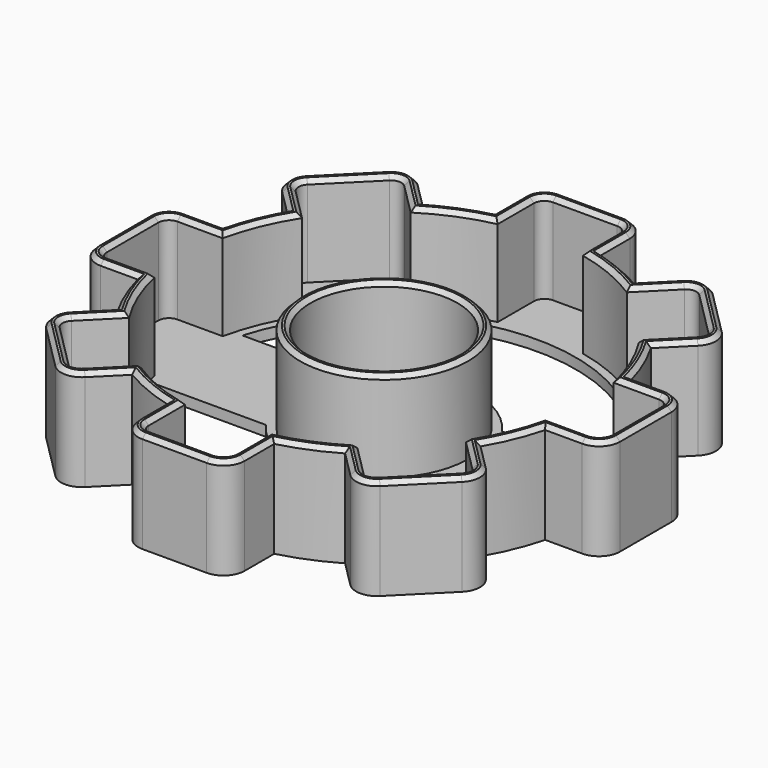
from build123d import *

# Parameters (mm, degrees)
F0_R     = 50.070430454
F0_R_2   = 17.4751749808
F2_DEPTH = 24
F3_COUNT = 8
F5_T     = -2.5
F6_SIZE  = 1
F8_DEPTH = 5


with BuildPart() as f2:
    # F0 (on Top) → F2 (new body)
    with BuildSketch(Plane.XY):
        with Locations((-6.849264726, -8.4674051031)):
            Circle(F0_R)
        with Locations((-6.849264726, -8.4674051031)):
            Circle(F0_R_2, mode=Mode.SUBTRACT)
    extrude(amount=F2_DEPTH)


with BuildPart() as f2b:
    # F1 (on Top) → F2, piece 2 (new body)
    with BuildSketch(Plane.XY):
        with BuildLine():
            Line((0.7983369527, 53.7766548421), (-14.4968664047, 53.7766548421))
            ThreePointArc((-14.4968664047, 53.7766548421), (-18.0324003107, 52.312188748), (-19.4968664047, 48.7766548421))
            Line((-19.4968664047, 48.7766548421), (-19.4968664047, 39.9793303661))
            Line((-19.4968664047, 39.9793303661), (5.7983369527, 39.9793303661))
            Line((5.7983369527, 39.9793303661), (5.7983369527, 48.7766548421))
            ThreePointArc((5.7983369527, 48.7766548421), (4.3338708586, 52.312188748), (0.7983369527, 53.7766548421))
        make_face()
    extrude(amount=F2_DEPTH)


with BuildPart() as f3_1:
    # F3: instance of F2b
    add(f2b.part.rotate(Axis((-6.849264726, -8.4674051031, 0), (0, 0, 1)), 1 * 360 / F3_COUNT))


with BuildPart() as f3_2:
    # F3: instance of F2b
    add(f2b.part.rotate(Axis((-6.849264726, -8.4674051031, 0), (0, 0, 1)), 2 * 360 / F3_COUNT))


with BuildPart() as f3_3:
    # F3: instance of F2b
    add(f2b.part.rotate(Axis((-6.849264726, -8.4674051031, 0), (0, 0, 1)), 3 * 360 / F3_COUNT))


with BuildPart() as f3_4:
    # F3: instance of F2b
    add(f2b.part.rotate(Axis((-6.849264726, -8.4674051031, 0), (0, 0, 1)), 4 * 360 / F3_COUNT))


with BuildPart() as f3_5:
    # F3: instance of F2b
    add(f2b.part.rotate(Axis((-6.849264726, -8.4674051031, 0), (0, 0, 1)), 5 * 360 / F3_COUNT))


with BuildPart() as f3_6:
    # F3: instance of F2b
    add(f2b.part.rotate(Axis((-6.849264726, -8.4674051031, 0), (0, 0, 1)), 6 * 360 / F3_COUNT))


with BuildPart() as f3_7:
    # F3: instance of F2b
    add(f2b.part.rotate(Axis((-6.849264726, -8.4674051031, 0), (0, 0, 1)), 7 * 360 / F3_COUNT))


with BuildPart() as f2b_1:
    add(f2b.part)

    # F4: union F3_7, F3_6, F3_5, F3_4, F3_3, F3_2, F3_1, F2
    add(f3_7.part)
    add(f3_6.part)
    add(f3_5.part)
    add(f3_4.part)
    add(f3_3.part)
    add(f3_2.part)
    add(f3_1.part)
    add(f2.part)

    # F5
    f5_openings = [f2b_1.faces().sort_by_distance(p)[0] for p in [
        (3.08899, 51.067308, 24),
    ]]
    offset(amount=F5_T, openings=f5_openings, kind=Kind.INTERSECTION)

    # F6
    f6_edges = [f2b_1.edges().sort_by_distance(p)[0] for p in [
        (-24.32444, -8.467405, 24),
        (-26.82444, -8.467405, 24),
        (4.333871, 52.312189, 24),
        (-6.849265, 53.776655, 24),
        (-18.0324, 52.312189, 24),
        (-19.496866, 44.377993, 24),
        (-26.010389, 37.791641, 24),
        (-35.273399, 37.843139, 24),
        (-41.919257, 42.417929, 24),
        (-50.862462, 35.545792, 24),
        (-57.734599, 26.602587, 24),
        (-53.159809, 19.956729, 24),
        (-53.108311, 10.693719, 24),
        (-59.694662, 4.180197, 24),
        (-67.628859, 2.71573, 24),
        (-69.093325, -8.467405, 24),
        (-67.628859, -19.650541, 24),
        (-59.694662, -21.115007, 24),
        (-53.108311, -27.628529, 24),
        (-53.159809, -36.891539, 24),
        (-57.734599, -43.537397, 24),
        (-50.862462, -52.480602, 24),
        (-41.919257, -59.352739, 24),
        (-35.273399, -54.777949, 24),
        (-26.010389, -54.726451, 24),
        (-19.496866, -61.312803, 24),
        (-18.0324, -69.246999, 24),
        (-6.849265, -70.711465, 24),
        (4.333871, -69.246999, 24),
        (5.798337, -61.312803, 24),
        (12.311859, -54.726451, 24),
        (21.574869, -54.777949, 24),
        (28.220727, -59.352739, 24),
        (37.163932, -52.480602, 24),
        (44.036069, -43.537397, 24),
        (39.461279, -36.891539, 24),
        (39.409781, -27.628529, 24),
        (45.996133, -21.115007, 24),
        (53.930329, -19.650541, 24),
        (55.394795, -8.467405, 24),
        (53.930329, 2.71573, 24),
        (45.996133, 4.180197, 24),
        (39.409781, 10.693719, 24),
        (39.461279, 19.956729, 24),
        (44.036069, 26.602587, 24),
        (37.163932, 35.545792, 24),
        (28.220727, 42.417929, 24),
        (21.574869, 37.843139, 24),
        (12.311859, 37.791641, 24),
        (5.798337, 44.377993, 24),
        (2.566104, 50.544422, 24),
        (3.298337, 43.392375, 24),
        (11.355151, 35.481942, 24),
        (22.645699, 35.378435, 24),
        (28.220727, 39.917929, 24),
        (35.396165, 33.778025, 24),
        (41.536069, 26.602587, 24),
        (36.996575, 21.027559, 24),
        (37.100082, 9.737011, 24),
        (45.010515, 1.680197, 24),
        (52.162562, 0.947964, 24),
        (52.894795, -8.467405, 24),
        (52.162562, -17.882774, 24),
        (45.010515, -18.615007, 24),
        (37.100082, -26.671821, 24),
        (36.996575, -37.962369, 24),
        (41.536069, -43.537397, 24),
        (35.396165, -50.712835, 24),
        (28.220727, -56.852739, 24),
        (22.645699, -52.313245, 24),
        (11.355151, -52.416752, 24),
        (3.298337, -60.327185, 24),
        (2.566104, -67.479232, 24),
        (-6.849265, -68.211465, 24),
        (-16.264633, -67.479232, 24),
        (-16.996866, -60.327185, 24),
        (-25.05368, -52.416752, 24),
        (-36.344229, -52.313245, 24),
        (-41.919257, -56.852739, 24),
        (-49.094695, -50.712835, 24),
        (-55.234599, -43.537397, 24),
        (-50.695105, -37.962369, 24),
        (-50.798612, -26.671821, 24),
        (-58.709044, -18.615007, 24),
        (-65.861092, -17.882774, 24),
        (-66.593325, -8.467405, 24),
        (-65.861092, 0.947964, 24),
        (-58.709044, 1.680197, 24),
        (-50.798612, 9.737011, 24),
        (-50.695105, 21.027559, 24),
        (-55.234599, 26.602587, 24),
        (-49.094695, 33.778025, 24),
        (-41.919257, 39.917929, 24),
        (-36.344229, 35.378435, 24),
        (-25.05368, 35.481942, 24),
        (-16.996866, 43.392375, 24),
        (-16.264633, 50.544422, 24),
        (-6.849265, 51.276655, 24),
    ]]
    chamfer(f6_edges, length=F6_SIZE)

    # F7 (on face) → F8 (cut)
    with BuildSketch(Plane.XY):
        with BuildLine():
            Line((-24.7759111502, -21.1450022194), (-50.6402311933, -21.1450022194))
            ThreePointArc((-50.6402311933, -21.1450022194), (-6.849264726, -54.0565508812), (36.9417017412, -21.1450022194))
            Line((36.9417017412, -21.1450022194), (11.0773816981, -21.1450022194))
            ThreePointArc((11.0773816981, -21.1450022194), (-6.849264726, -30.4238647599), (-24.7759111502, -21.1450022194))
        make_face()
        with BuildLine():
            ThreePointArc((36.9417017412, 4.2101920131), (-6.849264726, 37.1217406749), (-50.6402311933, 4.2101920131))
            Line((-50.6402311933, 4.2101920131), (-24.7759111502, 4.2101920131))
            ThreePointArc((-24.7759111502, 4.2101920131), (-6.849264726, 13.4890545536), (11.0773816981, 4.2101920131))
            Line((11.0773816981, 4.2101920131), (36.9417017412, 4.2101920131))
        make_face()
    extrude(amount=F8_DEPTH, mode=Mode.SUBTRACT)


solid = f2b_1.part
